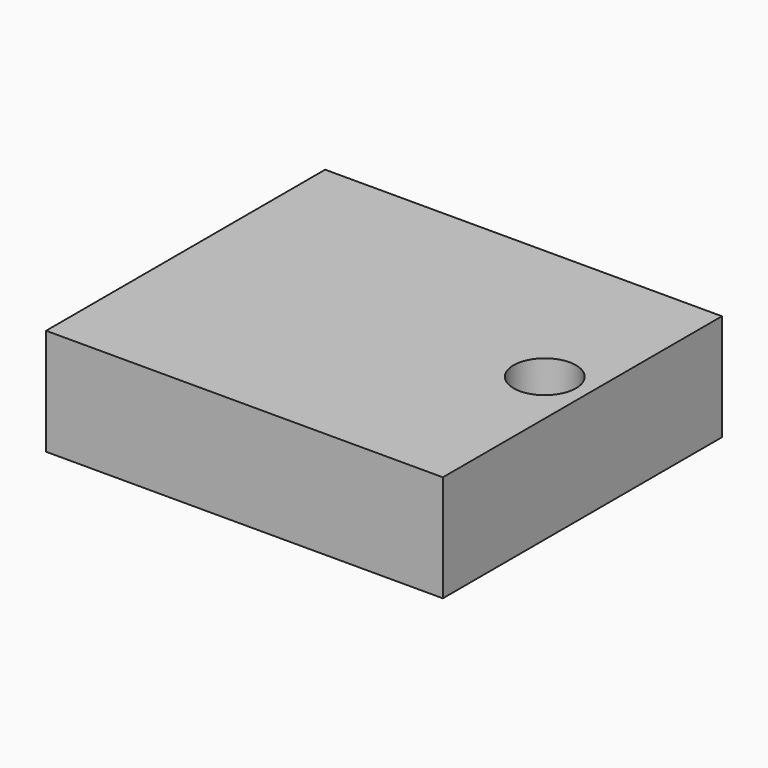
from build123d import *

# Parameters (mm, degrees)
F0_W     = 46.4574210346
F0_H     = 83.1440314651
F0_W_2   = 48.1166169047
F0_R     = 7.4407213522
F1_DEPTH = 25.4


with BuildPart() as f1:
    # F0 (on Top) → F1 (new body)
    with BuildSketch(Plane.XY):
        with Locations((-23.2287105173, -1.935724169)):
            Rectangle(F0_W, F0_H)
        with Locations((24.0583084524, -1.935724169)):
            Rectangle(F0_W_2, F0_H)
        with Locations((37.6083850861, 0)):
            Circle(F0_R, mode=Mode.SUBTRACT)
    extrude(amount=F1_DEPTH)


solid = f1.part
